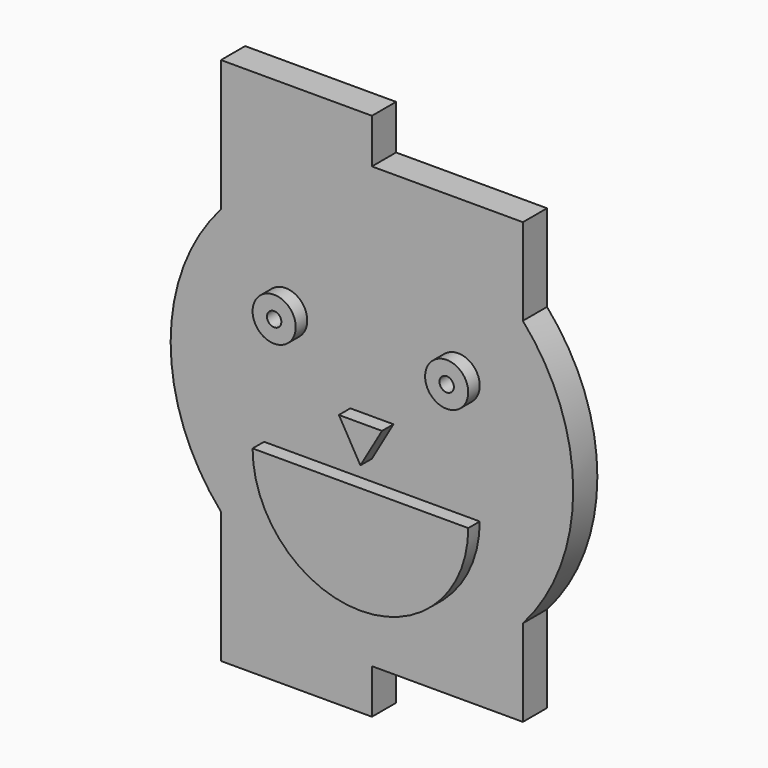
from build123d import *

# Parameters (mm, degrees)
F1_DEPTH = 2.1
F4_DEPTH = 1
F7_DEPTH = 1
F2_R     = 1.5
F2_R_2   = 0.5
F8_DEPTH = 1


# Not quite as in the source:
# - a feature names something its author has since deleted; it is built from what else it names
# - the program builds the solid bodies; features that only make, move or delete a surface that nothing else refers to are left out


with BuildPart() as f1:
    # F0 (on Front) → F1 (new body)
    with BuildSketch(Plane.XZ):
        with BuildLine():
            ThreePointArc((-10.5, 9.2601295887), (-14, 0), (-10.5, -9.2601295887))
            Line((-10.5, -9.2601295887), (-10.5, -18.4))
            Line((-10.5, -18.4), (0, -18.4))
            Line((0, -18.4), (0, -15.3))
            Line((0, -15.3), (10.5, -15.3))
            Line((10.5, -15.3), (10.5, -9.2601295887))
            ThreePointArc((10.5, -9.2601295887), (14, 0), (10.5, 9.2601295887))
            Line((10.5, 9.2601295887), (10.5, 15.3))
            Line((10.5, 15.3), (0, 15.3))
            Line((0, 15.3), (0, 18.4))
            Line((0, 18.4), (-10.5, 18.4))
            Line((-10.5, 18.4), (-10.5, 9.2601295887))
        make_face()
    extrude(amount=-F1_DEPTH)

    # F3 (on face) → F4 (join)
    with BuildSketch(Plane.XZ):
        Polygon((1.5, 0), (-1.5, 0), (0, -2.5980762114), align=None)
    extrude(amount=F4_DEPTH)

    # F5 (on face) → F7 (join)
    with BuildSketch(Plane.XZ):
        with BuildLine():
            Line((0, -4), (-7.5, -4))
            ThreePointArc((-7.5, -4), (0, -11.5), (7.5, -4))
            Line((7.5, -4), (0, -4))
        make_face()
    extrude(amount=F7_DEPTH)

    # F2 (on Front) → F8 (join)
    with BuildSketch(Plane.XZ):
        with Locations((-6, 4.4)):
            Circle(F2_R)
        with Locations((-6, 4.4)):
            Circle(F2_R_2, mode=Mode.SUBTRACT)
        with Locations((5.9996811691, 4.3125251973)):
            Circle(F2_R)
        with Locations((5.9996811691, 4.3125251973)):
            Circle(F2_R_2, mode=Mode.SUBTRACT)
    extrude(amount=F8_DEPTH)


solid = f1.part
